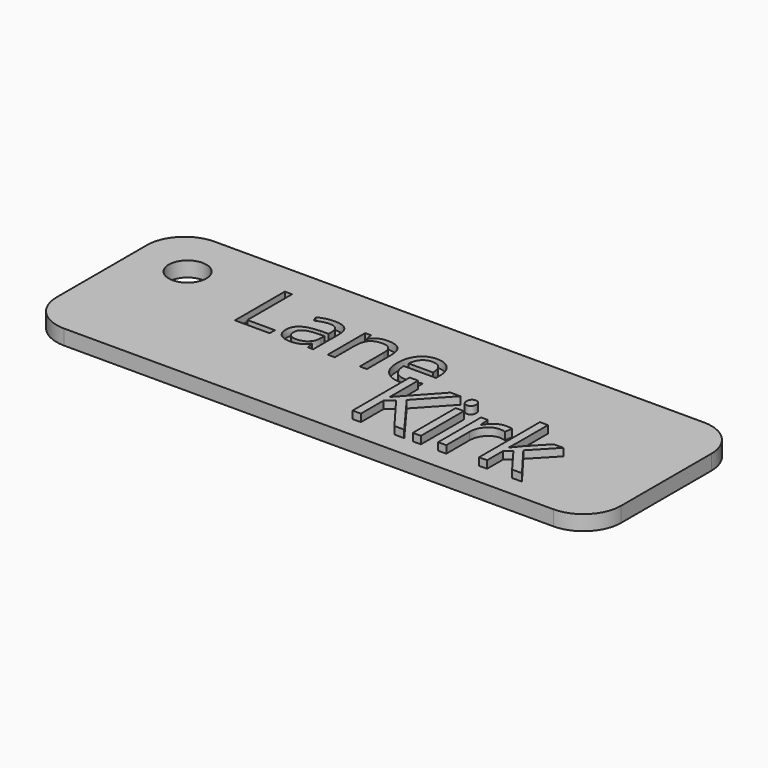
from build123d import *

# Parameters (mm, degrees)
F1_DEPTH     = 2
F3_D         = 5
F4_TEXT_SIZE = 11.6051963737
F5_DEPTH     = 1
F6_TEXT_SIZE = 13.3056467575
F7_DEPTH     = 1


# Not quite as in the source:
# - Text() gives the source's letters only with a copy of the font that has no kerning and outlines rounded to 1/6400 em; it was checked with that copy


with BuildPart() as f1:
    # F0 (on Top) → F1 (new body)
    with BuildSketch(Plane.XY):
        with BuildLine():
            ThreePointArc((37.5, 7.5), (36.0355339059, 11.0355339059), (32.5, 12.5))
            Line((32.5, 12.5), (-32.5, 12.5))
            ThreePointArc((-32.5, 12.5), (-36.0355339059, 11.0355339059), (-37.5, 7.5))
            Line((-37.5, 7.5), (-37.5, -7.5))
            ThreePointArc((-37.5, -7.5), (-36.0355339059, -11.0355339059), (-32.5, -12.5))
            Line((-32.5, -12.5), (32.5, -12.5))
            ThreePointArc((32.5, -12.5), (36.0355339059, -11.0355339059), (37.5, -7.5))
            Line((37.5, -7.5), (37.5, 7.5))
        make_face()
    extrude(amount=F1_DEPTH)

    # F3 (through all)
    with Locations(Plane.XY.offset(2)):
        with Locations((-30.5, 5.5)):
            Hole(F3_D / 2)

    # F4 (on face) → F5 (cut)
    with BuildSketch(Plane.XY.offset(2)):
        with Locations((-20.9465846419, 0)):
            Text('Lane', F4_TEXT_SIZE, font='Open Sans', text_align=(TextAlign.LEFT, TextAlign.BOTTOM))
    extrude(amount=-F5_DEPTH, mode=Mode.SUBTRACT)

    # F6 (on face) → F7 (join)
    with BuildSketch(Plane.XY.offset(2)):
        with Locations((2.2746879772, -9.6943043172)):
            Text('Kirk', F6_TEXT_SIZE, font='Open Sans', text_align=(TextAlign.LEFT, TextAlign.BOTTOM))
    extrude(amount=F7_DEPTH)


solid = f1.part
